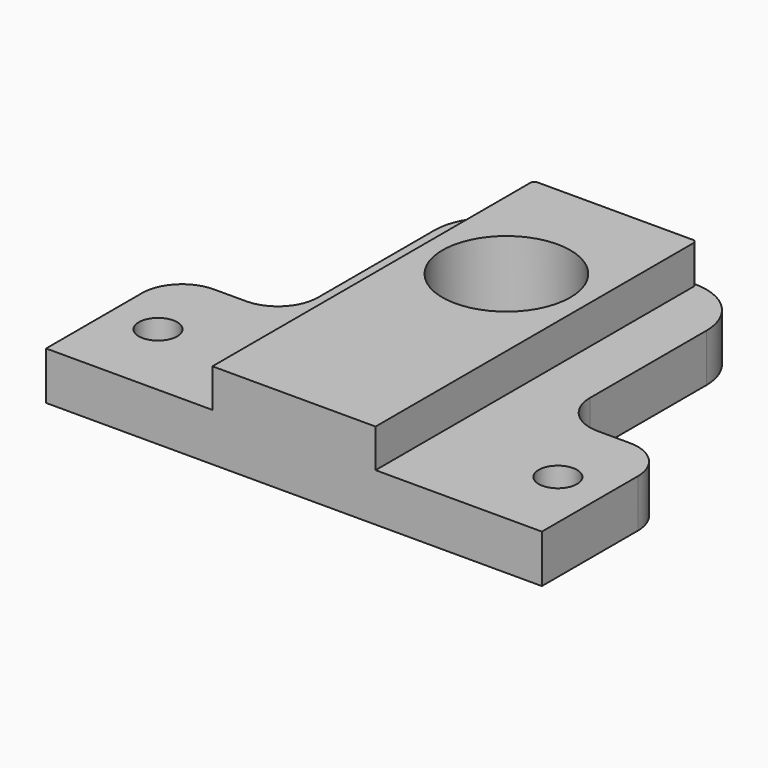
from build123d import *

# Parameters (mm, degrees)
F1_DEPTH     = 6
F2_W         = 20.4
F2_H         = 50.2
F3_DEPTH     = 4.8
F4_R         = 8
F5_DEPTH     = 10.801
F6_R         = 2.4
F7_DEPTH     = 6.001
F8_R         = 7
F9_R         = 5
F10_T1_DEPTH = 6.0500204163


# Not quite as in the source:
# - a fillet or chamfer that OpenCascade refuses, or shapes differently, is made with other operations: its cross-section is extruded or revolved along the edge and cut away or added


with BuildPart() as f1:
    # F0 (on Top) → F1 (new body)
    with BuildSketch(Plane.XY):
        Polygon((-31, 20), (-31, 0), (31, 0), (31, 20), (17, 20), (17, 50.2), (-17, 50.2), (-17, 20), align=None)
    extrude(amount=F1_DEPTH)

    # F2 (on face) → F3 (join)
    with BuildSketch(Plane.XY.offset(6)):
        with Locations((0, 25.1)):
            Rectangle(F2_W, F2_H)
    extrude(amount=F3_DEPTH)

    # F4 (on face) → F5 (cut, through all)
    with BuildSketch(Plane.XY.offset(10.8)):
        with Locations((0, 33.2)):
            Circle(F4_R)
    extrude(amount=-F5_DEPTH, mode=Mode.SUBTRACT)

    # F6 (on face) → F7 (cut, through all)
    with BuildSketch(Plane.XY.offset(6)):
        with Locations((-25, 10)):
            Circle(F6_R)
        with Locations((25, 10)):
            Circle(F6_R)
    extrude(amount=-F7_DEPTH, mode=Mode.SUBTRACT)

    # F8
    f8_edges = [f1.edges().sort_by_distance(p)[0] for p in [
        (17, 50.2, 3),
        (-17, 50.2, 3),
    ]]
    fillet(f8_edges, radius=F8_R)

    # F9
    f9_edges = [f1.edges().sort_by_distance(p)[0] for p in [
        (-31, 20, 3),
        (31, 20, 3),
        (17, 20, 3),
        (-17, 20, 3),
    ]]
    fillet(f9_edges, radius=F9_R)

    # F10: fillet of radius 0.5 on 2 edges, made by hand

    # F10_s2 → F10_t1 (cut)
    with BuildSketch(Plane.XY.offset(6)):
        with BuildLine():
            ThreePointArc((9.7, 50.2), (10.0535533906, 50.0535533906), (10.2, 49.7))
            Line((10.2, 49.7), (10.25, 49.7))
            Line((10.25, 49.7), (10.25, 50.1971422738))
            Line((10.25, 50.1971422738), (10.2014285714, 50.2471218615))
            ThreePointArc((10.2014285714, 50.2471218615), (10, 50.25), (9.7, 50.25))
            Line((9.7, 50.25), (9.7, 50.2))
        make_face()
        with BuildLine():
            ThreePointArc((-9.7, 50.2), (-10.0535533906, 50.0535533906), (-10.2, 49.7))
            Line((-10.2, 49.7), (-10.25, 49.7))
            Line((-10.25, 49.7), (-10.25, 50.1971422738))
            Line((-10.25, 50.1971422738), (-10.2014285714, 50.2471218615))
            ThreePointArc((-10.2014285714, 50.2471218615), (-10, 50.25), (-9.7, 50.25))
            Line((-9.7, 50.25), (-9.7, 50.2))
        make_face()
    extrude(amount=F10_T1_DEPTH, mode=Mode.SUBTRACT)


solid = f1.part
